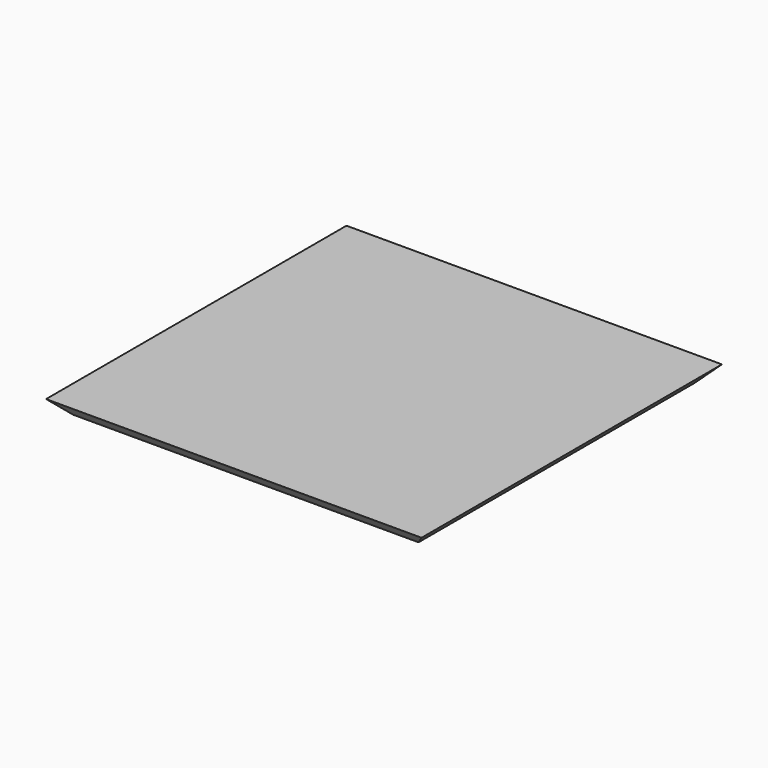
from build123d import *

# Parameters (mm, degrees)
F0_W     = 635
F0_H     = 635
F1_DEPTH = 25.4
F2_SIZE  = 25.39999


# Not quite as in the source:
# - a fillet or chamfer is up to 0.001 mm smaller than in the source, because OpenCascade refuses the exact size


with BuildPart() as f1:
    # F0 (on Top) → F1 (new body)
    with BuildSketch(Plane.XY):
        Rectangle(F0_W, F0_H)
    extrude(amount=F1_DEPTH)

    # F2 (size 25.4 in the source; OpenCascade refuses exactly that, so slightly less here)
    f2_edges = [f1.edges().sort_by_distance(p)[0] for p in [
        (0, 317.5, 0),
        (-317.5, 0, 0),
        (0, -317.5, 0),
        (317.5, 0, 0),
    ]]
    chamfer(f2_edges, length=F2_SIZE)


solid = f1.part
